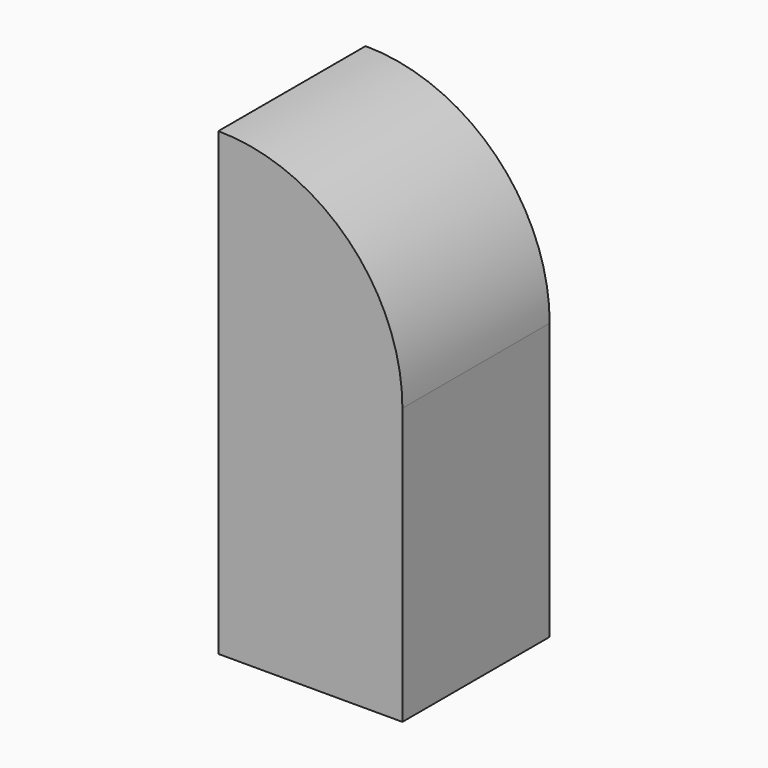
from build123d import *

# Parameters (mm, degrees)
F0_W     = 50.8
F0_H     = 50.8
F1_DEPTH = 63.5
F2_R     = 50.79999


# Not quite as in the source:
# - a fillet or chamfer is up to 0.001 mm smaller than in the source, because OpenCascade refuses the exact size


with BuildPart() as f1:
    # F0 (on Top) → F1 (new body, symmetric)
    with BuildSketch(Plane.XY):
        Rectangle(F0_W, F0_H)
    extrude(amount=F1_DEPTH, both=True)

    # F2 (radius 50.8 in the source; OpenCascade refuses exactly that, so slightly less here)
    f2_edges = [f1.edges().sort_by_distance(p)[0] for p in [
        (25.4, 0, 63.5),
    ]]
    fillet(f2_edges, radius=F2_R)


solid = f1.part
